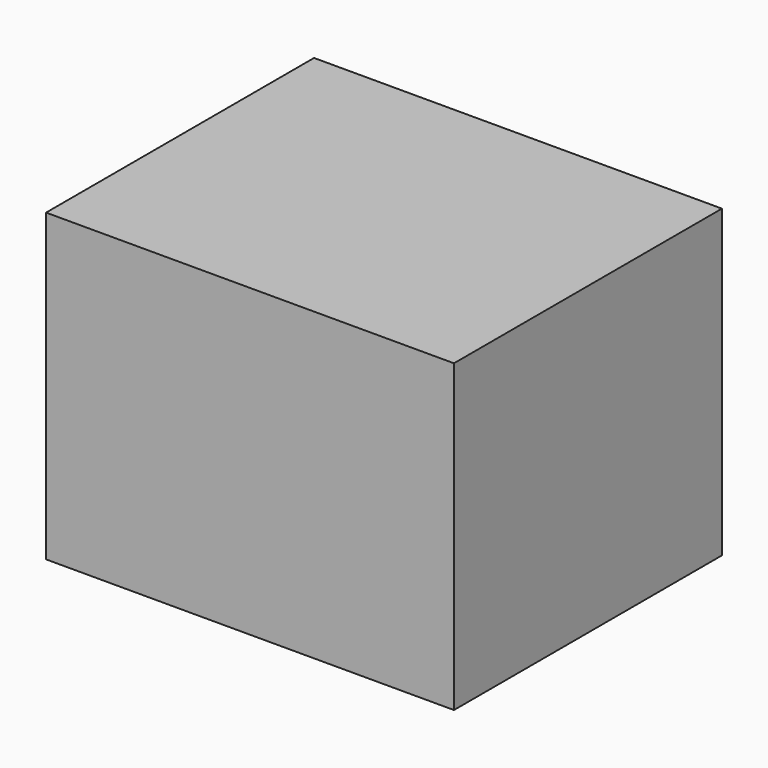
from build123d import *

# Parameters (mm, degrees)
F0_W     = 101.8076017499
F0_H     = 83.6001895368
F5_DEPTH = 76.2


# Not quite as in the source:
# - a feature of the source that left no trace in its solid (it failed there, or was rolled back) is left out


with BuildPart() as f5:
    # F0 (on Top) → F5 (new body)
    with BuildSketch(Plane.XY):
        with Locations((3.461971879, 1.0257679969)):
            Rectangle(F0_W, F0_H)
    extrude(amount=-F5_DEPTH)


solid = f5.part
